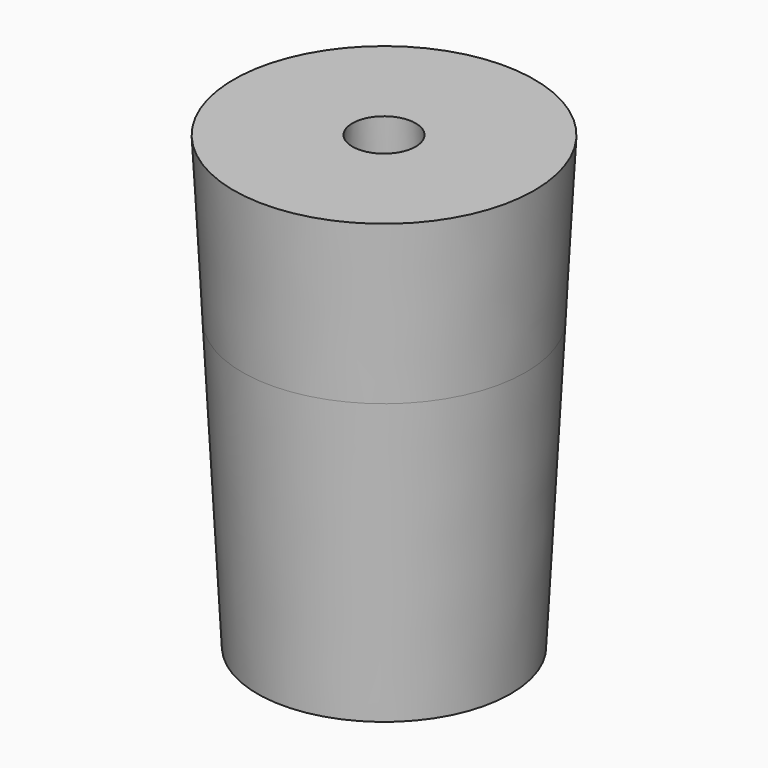
from build123d import *

# Parameters (mm, degrees)
F0_R        = 43.8484105158
F0_R_2      = 19.1409794654
F1_DEPTH    = 99.695
F1_TAPER    = -3
F1_FACE_R   = 49.0732040715
F1_FACE_R_2 = 13.9161859098
F2_DEPTH    = 56.388
F2_TAPER    = -3


# Not quite as in the source:
# - a feature of the source that left no trace in its solid (it failed there, or was rolled back) is left out


with BuildPart() as f1:
    # F0 (on Top) → F1 (new body)
    with BuildSketch(Plane.XY):
        with Locations((-177.5637567043, -11.3275945187)):
            Circle(F0_R)
        with Locations((-177.5637567043, -11.3275945187)):
            Circle(F0_R_2, mode=Mode.SUBTRACT)
    extrude(amount=F1_DEPTH, taper=F1_TAPER)

    # F1_face (on face) → F2 (join)
    with BuildSketch(Plane(origin=(-177.5637567043, -11.3275945187, 99.695), x_dir=(1, 0, 0), z_dir=(0, 0, 1))):
        Circle(F1_FACE_R)
        Circle(F1_FACE_R_2, mode=Mode.SUBTRACT)
    extrude(amount=F2_DEPTH, taper=F2_TAPER)


solid = f1.part
